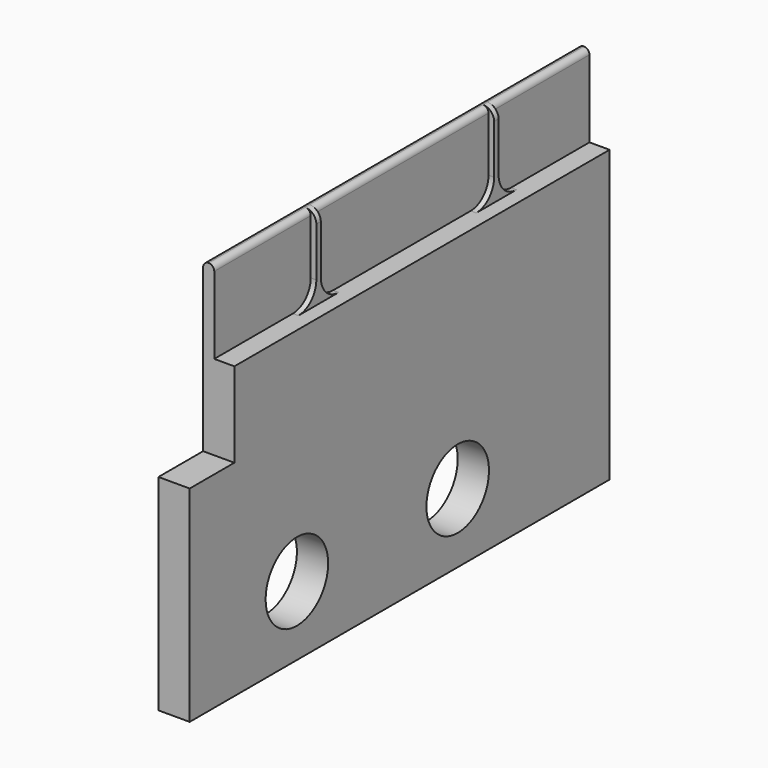
from build123d import *

# Parameters (mm, degrees)
F1_DEPTH = 1.4
F2_W     = 0.5
F2_H     = 21
F3_DEPTH = 3.7
F5_D     = 3.5
F7_DEPTH = 0.25
F8_R     = 0.24999
F9_R     = 0.4999


# Not quite as in the source:
# - a fillet or chamfer is up to 0.001 mm smaller than in the source, because OpenCascade refuses the exact size


with BuildPart() as f1:
    # F0 (on Right) → F1 (new body)
    with BuildSketch(Plane.YZ):
        Polygon((0, 9.2), (0, 0), (23.5, 0), (23.5, 13), (2.5, 13), (2.5, 9.2), align=None)
    extrude(amount=F1_DEPTH)

    # F2 (on face) → F3 (join)
    with BuildSketch(Plane.XY.offset(13)):
        with Locations((0.25, 13)):
            Rectangle(F2_W, F2_H)
    extrude(amount=F3_DEPTH)

    # F5 (through all)
    with Locations(Plane.YZ.offset(1.4)):
        with Locations((6, 3.1), (15, 3.1)):
            Hole(F5_D / 2)

    # F6 (on face) → F7 (join)
    with BuildSketch(Plane.YZ.offset(0.5)):
        with BuildLine():
            Line((7.9, 16.7), (7.9, 14))
            ThreePointArc((7.9, 14), (7.6071067812, 13.2928932188), (6.9, 13))
            Line((6.9, 13), (7.9, 13))
            Line((7.9, 13), (8.15, 13))
            Line((8.15, 13), (9.15, 13))
            ThreePointArc((9.15, 13), (8.4428932188, 13.2928932188), (8.15, 14))
            Line((8.15, 14), (8.15, 16.7))
            Line((8.15, 16.7), (7.9, 16.7))
        make_face()
        with BuildLine():
            Line((18.1, 16.7), (17.85, 16.7))
            Line((17.85, 16.7), (17.85, 14))
            ThreePointArc((17.85, 14), (17.5571067812, 13.2928932188), (16.85, 13))
            Line((16.85, 13), (17.85, 13))
            Line((17.85, 13), (18.1, 13))
            Line((18.1, 13), (19.1, 13))
            ThreePointArc((19.1, 13), (18.3928932188, 13.2928932188), (18.1, 14))
            Line((18.1, 14), (18.1, 16.7))
        make_face()
    extrude(amount=F7_DEPTH)

    # F8 (radius 0.25 in the source; OpenCascade refuses exactly that, so slightly less here)
    f8_edges = [f1.edges().sort_by_distance(p)[0] for p in [
        (0, 13, 16.7),
        (0.5, 20.8, 16.7),
        (0.5, 13, 16.7),
        (0.5, 5.2, 16.7),
    ]]
    fillet(f8_edges, radius=F8_R)

    # F9 (radius 0.5 in the source; OpenCascade refuses exactly that, so slightly less here)
    f9_edges = [f1.edges().sort_by_distance(p)[0] for p in [
        (0.75, 8.025, 16.7),
        (0.75, 17.975, 16.7),
    ]]
    fillet(f9_edges, radius=F9_R)


solid = f1.part
